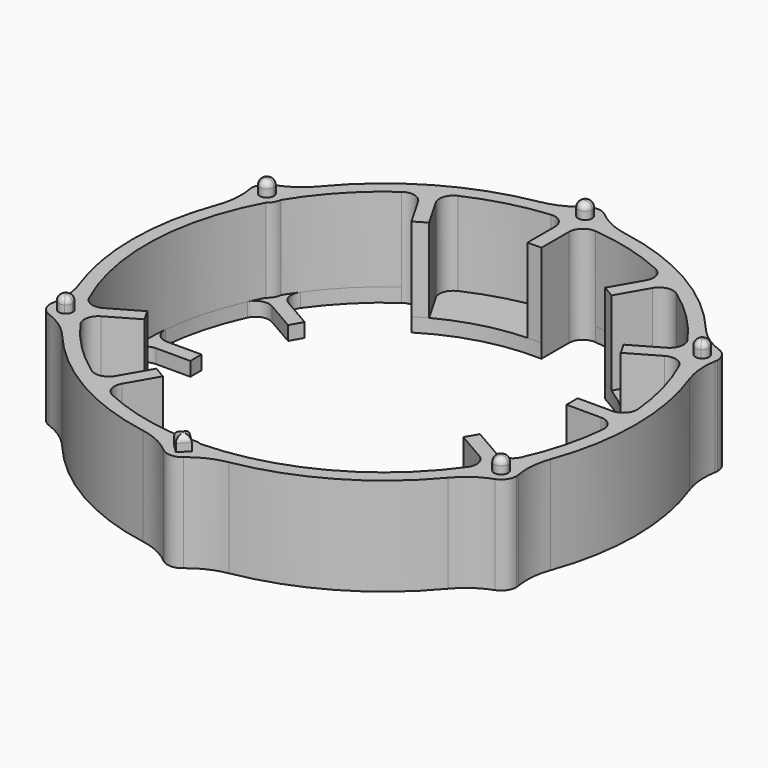
from build123d import *

# Parameters (mm, degrees)
F1_R         = 18
F1_R_2       = 17
F2_DEPTH     = 7
F3_DEPTH     = 7
F4_DEPTH     = 1
F6_DEPTH     = 7
F7_R         = 1
F8_R         = 5
F9_DEPTH     = 8
F10_R        = 0.44999
F11_DEPTH    = 1.8
F12_R        = 13.47
F13_DEPTH    = 1
F14_DEPTH    = 1
F15_T1_DEPTH = 1
F15_T3_DEPTH = 3.7395798703


# Not quite as in the source:
# - a fillet or chamfer that OpenCascade refuses, or shapes differently, is made with other operations: its cross-section is extruded or revolved along the edge and cut away or added
# - a fillet or chamfer is up to 0.001 mm smaller than in the source, because OpenCascade refuses the exact size


with BuildPart() as f2:
    # F1 (on Top) → F2 (new body)
    with BuildSketch(Plane.XY):
        Circle(F1_R)
        Circle(F1_R_2, mode=Mode.SUBTRACT)
    extrude(amount=F2_DEPTH)

    # F0 (on Top) → F3 (join)
    with BuildSketch(Plane.XY):
        with BuildLine():
            Line((7.1633711619, 11.4073228059), (8.9293354359, 14.4660626528))
            ThreePointArc((8.9293354359, 14.4660626528), (8.5, 14.7224318643), (8.0633100321, 14.9660626528))
            Line((8.0633100321, 14.9660626528), (6.2973457581, 11.9073228059))
            ThreePointArc((6.2973457581, 11.9073228059), (6.735, 11.665362189), (7.1633711619, 11.4073228059))
        make_face()
        with BuildLine():
            ThreePointArc((17, 0), (16.9981612676, 0.2500270431), (16.992645468, 0.5))
            Line((16.992645468, 0.5), (13.46071692, 0.5))
            ThreePointArc((13.46071692, 0.5), (13.46767903, 0.2500430841), (13.47, 0))
            ThreePointArc((13.47, 0), (13.46767903, -0.2500430841), (13.46071692, -0.5))
            Line((13.46071692, -0.5), (16.992645468, -0.5))
            ThreePointArc((16.992645468, -0.5), (16.9981612676, -0.2500270431), (17, 0))
        make_face()
        with BuildLine():
            ThreePointArc((-14.9660626528, -8.0633100321), (-14.7224318643, -8.5), (-14.4660626528, -8.9293354359))
            Line((-14.4660626528, -8.9293354359), (-11.4073228059, -7.1633711619))
            ThreePointArc((-11.4073228059, -7.1633711619), (-11.665362189, -6.735), (-11.9073228059, -6.2973457581))
            Line((-11.9073228059, -6.2973457581), (-14.9660626528, -8.0633100321))
        make_face()
        with BuildLine():
            Line((-6.2973457581, 11.9073228059), (-8.0633100321, 14.9660626528))
            ThreePointArc((-8.0633100321, 14.9660626528), (-8.5, 14.7224318643), (-8.9293354359, 14.4660626528))
            Line((-8.9293354359, 14.4660626528), (-7.1633711619, 11.4073228059))
            ThreePointArc((-7.1633711619, 11.4073228059), (-6.735, 11.665362189), (-6.2973457581, 11.9073228059))
        make_face()
        with BuildLine():
            Line((0.5, 13.46071692), (0.5, 16.992645468))
            ThreePointArc((0.5, 16.992645468), (0, 17), (-0.5, 16.992645468))
            Line((-0.5, 16.992645468), (-0.5, 13.46071692))
            ThreePointArc((-0.5, 13.46071692), (0, 13.47), (0.5, 13.46071692))
        make_face()
        with BuildLine():
            Line((11.9073228059, 6.2973457581), (14.9660626528, 8.0633100321))
            ThreePointArc((14.9660626528, 8.0633100321), (14.7224318643, 8.5), (14.4660626528, 8.9293354359))
            Line((14.4660626528, 8.9293354359), (11.4073228059, 7.1633711619))
            ThreePointArc((11.4073228059, 7.1633711619), (11.665362189, 6.735), (11.9073228059, 6.2973457581))
        make_face()
        with BuildLine():
            ThreePointArc((14.4660626528, -8.9293354359), (14.7224318643, -8.5), (14.9660626528, -8.0633100321))
            Line((14.9660626528, -8.0633100321), (11.9073228059, -6.2973457581))
            ThreePointArc((11.9073228059, -6.2973457581), (11.665362189, -6.735), (11.4073228059, -7.1633711619))
            Line((11.4073228059, -7.1633711619), (14.4660626528, -8.9293354359))
        make_face()
        with BuildLine():
            ThreePointArc((-8.9293354359, -14.4660626528), (-8.5, -14.7224318643), (-8.0633100321, -14.9660626528))
            Line((-8.0633100321, -14.9660626528), (-6.2973457581, -11.9073228059))
            ThreePointArc((-6.2973457581, -11.9073228059), (-6.735, -11.665362189), (-7.1633711619, -11.4073228059))
            Line((-7.1633711619, -11.4073228059), (-8.9293354359, -14.4660626528))
        make_face()
    extrude(amount=F3_DEPTH)

    # F1 (on Top) → F4 (join)
    with BuildSketch(Plane.XY):
        Circle(F1_R)
        Circle(F1_R_2, mode=Mode.SUBTRACT)
        Circle(F1_R_2)
    extrude(amount=F4_DEPTH)

    # F5 (on Top) → F6 (join)
    with BuildSketch(Plane.XY):
        with BuildLine():
            ThreePointArc((-14.4884572681, 9), (-14.6275367743, 9.5353800561), (-15.0096060035, 9.935377578))
            ThreePointArc((-15.0096060035, 9.935377578), (-15.1731450826, 9.6837837802), (-15.3324673166, 9.4294987133))
            ThreePointArc((-15.3324673166, 9.4294987133), (-15.153718855, 9.2469868663), (-15.0884572681, 9))
            ThreePointArc((-15.0884572681, 9), (-15.3354561915, 8.5687338928), (-15.832419089, 8.5635568422))
            ThreePointArc((-15.832419089, 8.5635568422), (-15.9729752997, 8.2984372068), (-16.1090923805, 8.0310113108))
            ThreePointArc((-16.1090923805, 8.0310113108), (-15.0239657375, 8.0558870238), (-14.4884572681, 9))
        make_face()
        with BuildLine():
            ThreePointArc((-15.3324673166, 9.4294987133), (-15.1731450826, 9.6837837802), (-15.0096060035, 9.935377578))
            ThreePointArc((-15.0096060035, 9.935377578), (-16.5410852123, 9.55), (-16.1090923805, 8.0310113108))
            ThreePointArc((-16.1090923805, 8.0310113108), (-15.9729752997, 8.2984372068), (-15.832419089, 8.5635568422))
            ThreePointArc((-15.832419089, 8.5635568422), (-16.02146997, 9.25), (-15.3324673166, 9.4294987133))
        make_face()
        with BuildLine():
            ThreePointArc((-1.099486377, 17.9663888889), (0, 16.9), (1.099486377, 17.9663888889))
            ThreePointArc((1.099486377, 17.9663888889), (0.7998302171, 17.982220987), (0.4999517724, 17.9930555556))
            ThreePointArc((0.4999517724, 17.9930555556), (0, 17.5), (-0.4999517724, 17.9930555556))
            ThreePointArc((-0.4999517724, 17.9930555556), (-0.7998302171, 17.982220987), (-1.099486377, 17.9663888889))
        make_face()
        with BuildLine():
            ThreePointArc((0.4999517724, 17.9930555556), (0.7998302171, 17.982220987), (1.099486377, 17.9663888889))
            ThreePointArc((1.099486377, 17.9663888889), (1.0998715868, 17.9831924823), (1.1, 18))
            ThreePointArc((1.1, 18), (-0.0168075177, 19.0998715868), (-1.099486377, 17.9663888889))
            ThreePointArc((-1.099486377, 17.9663888889), (-0.7998302171, 17.982220987), (-0.4999517724, 17.9930555556))
            ThreePointArc((-0.4999517724, 17.9930555556), (-0.003472306, 18.4999879429), (0.5, 18))
            ThreePointArc((0.5, 18), (0.4999879429, 17.996527694), (0.4999517724, 17.9930555556))
        make_face()
        with BuildLine():
            ThreePointArc((15.832419089, 8.5635568422), (15.9729752997, 8.2984372068), (16.1090923805, 8.0310113108))
            ThreePointArc((16.1090923805, 8.0310113108), (16.5325702443, 8.4355084694), (16.6884572681, 9))
            ThreePointArc((16.6884572681, 9), (16.1238373242, 9.9609204939), (15.0096060035, 9.935377578))
            ThreePointArc((15.0096060035, 9.935377578), (15.1731450826, 9.6837837802), (15.3324673166, 9.4294987133))
            ThreePointArc((15.3324673166, 9.4294987133), (15.8354441344, 9.4347384132), (16.0884572681, 9))
            ThreePointArc((16.0884572681, 9), (16.0197233753, 8.7469989234), (15.832419089, 8.5635568422))
        make_face()
        with BuildLine():
            ThreePointArc((15.0096060035, 9.935377578), (14.635829324, 8.45), (16.1090923805, 8.0310113108))
            ThreePointArc((16.1090923805, 8.0310113108), (15.9729752997, 8.2984372068), (15.832419089, 8.5635568422))
            ThreePointArc((15.832419089, 8.5635568422), (15.1554445662, 8.75), (15.3324673166, 9.4294987133))
            ThreePointArc((15.3324673166, 9.4294987133), (15.1731450826, 9.6837837802), (15.0096060035, 9.935377578))
        make_face()
        with BuildLine():
            ThreePointArc((-15.3324673166, -9.4294987133), (-15.1731450826, -9.6837837802), (-15.0096060035, -9.935377578))
            ThreePointArc((-15.0096060035, -9.935377578), (-14.6275367743, -9.5353800561), (-14.4884572681, -9))
            ThreePointArc((-14.4884572681, -9), (-15.0239657375, -8.0558870238), (-16.1090923805, -8.0310113108))
            ThreePointArc((-16.1090923805, -8.0310113108), (-15.9729752997, -8.2984372068), (-15.832419089, -8.5635568422))
            ThreePointArc((-15.832419089, -8.5635568422), (-15.3354561915, -8.5687338928), (-15.0884572681, -9))
            ThreePointArc((-15.0884572681, -9), (-15.153718855, -9.2469868663), (-15.3324673166, -9.4294987133))
        make_face()
        with BuildLine():
            ThreePointArc((-16.1090923805, -8.0310113108), (-16.5410852123, -9.55), (-15.0096060035, -9.935377578))
            ThreePointArc((-15.0096060035, -9.935377578), (-15.1731450826, -9.6837837802), (-15.3324673166, -9.4294987133))
            ThreePointArc((-15.3324673166, -9.4294987133), (-16.02146997, -9.25), (-15.832419089, -8.5635568422))
            ThreePointArc((-15.832419089, -8.5635568422), (-15.9729752997, -8.2984372068), (-16.1090923805, -8.0310113108))
        make_face()
        with BuildLine():
            ThreePointArc((0.6255239257, -17.9891278226), (0.8625800837, -17.9793202207), (1.099486377, -17.9663888889))
            ThreePointArc((1.099486377, -17.9663888889), (0, -16.9), (-1.099486377, -17.9663888889))
            ThreePointArc((-1.099486377, -17.9663888889), (-0.8625800837, -17.9793202207), (-0.6255239257, -17.9891278226))
            Line((-0.6255239257, -17.9891278226), (0, -17.3636038969))
            Line((0, -17.3636038969), (0.6255239257, -17.9891278226))
        make_face()
        with BuildLine():
            ThreePointArc((1.1, -18), (1.0998715868, -17.9831924823), (1.099486377, -17.9663888889))
            ThreePointArc((1.099486377, -17.9663888889), (0.8625800837, -17.9793202207), (0.6255239257, -17.9891278226))
            Line((0.6255239257, -17.9891278226), (0.6363961031, -18))
            Line((0.6363961031, -18), (0, -18.6363961031))
            Line((0, -18.6363961031), (-0.6363961031, -18))
            Line((-0.6363961031, -18), (-0.6255239257, -17.9891278226))
            ThreePointArc((-0.6255239257, -17.9891278226), (-0.8625800837, -17.9793202207), (-1.099486377, -17.9663888889))
            ThreePointArc((-1.099486377, -17.9663888889), (-0.0168075177, -19.0998715868), (1.1, -18))
        make_face()
        with BuildLine():
            ThreePointArc((16.6884572681, -9), (16.5325702443, -8.4355084694), (16.1090923805, -8.0310113108))
            ThreePointArc((16.1090923805, -8.0310113108), (15.9729752997, -8.2984372068), (15.832419089, -8.5635568422))
            ThreePointArc((15.832419089, -8.5635568422), (16.0197233753, -8.7469989234), (16.0884572681, -9))
            ThreePointArc((16.0884572681, -9), (15.8354441344, -9.4347384132), (15.3324673166, -9.4294987133))
            ThreePointArc((15.3324673166, -9.4294987133), (15.1731450826, -9.6837837802), (15.0096060035, -9.935377578))
            ThreePointArc((15.0096060035, -9.935377578), (16.1238373242, -9.9609204939), (16.6884572681, -9))
        make_face()
        with BuildLine():
            ThreePointArc((15.832419089, -8.5635568422), (15.9729752997, -8.2984372068), (16.1090923805, -8.0310113108))
            ThreePointArc((16.1090923805, -8.0310113108), (14.635829324, -8.45), (15.0096060035, -9.935377578))
            ThreePointArc((15.0096060035, -9.935377578), (15.1731450826, -9.6837837802), (15.3324673166, -9.4294987133))
            ThreePointArc((15.3324673166, -9.4294987133), (15.1554445662, -8.75), (15.832419089, -8.5635568422))
        make_face()
        with BuildLine():
            ThreePointArc((-15.0884572681, 9), (-15.153718855, 9.2469868663), (-15.3324673166, 9.4294987133))
            ThreePointArc((-15.3324673166, 9.4294987133), (-15.5884572681, 9), (-15.832419089, 8.5635568422))
            ThreePointArc((-15.832419089, 8.5635568422), (-15.3354561915, 8.5687338928), (-15.0884572681, 9))
        make_face()
        with BuildLine():
            ThreePointArc((-15.832419089, 8.5635568422), (-15.5884572681, 9), (-15.3324673166, 9.4294987133))
            ThreePointArc((-15.3324673166, 9.4294987133), (-16.02146997, 9.25), (-15.832419089, 8.5635568422))
        make_face()
        with BuildLine():
            ThreePointArc((-0.4999517724, 17.9930555556), (0, 18), (0.4999517724, 17.9930555556))
            ThreePointArc((0.4999517724, 17.9930555556), (0.4999879429, 17.996527694), (0.5, 18))
            ThreePointArc((0.5, 18), (-0.003472306, 18.4999879429), (-0.4999517724, 17.9930555556))
        make_face()
        with BuildLine():
            ThreePointArc((-0.4999517724, 17.9930555556), (0, 17.5), (0.4999517724, 17.9930555556))
            ThreePointArc((0.4999517724, 17.9930555556), (0, 18), (-0.4999517724, 17.9930555556))
        make_face()
        with BuildLine():
            ThreePointArc((15.3324673166, 9.4294987133), (15.5884572681, 9), (15.832419089, 8.5635568422))
            ThreePointArc((15.832419089, 8.5635568422), (16.0197233753, 8.7469989234), (16.0884572681, 9))
            ThreePointArc((16.0884572681, 9), (15.8354441344, 9.4347384132), (15.3324673166, 9.4294987133))
        make_face()
        with BuildLine():
            ThreePointArc((15.3324673166, 9.4294987133), (15.1554445662, 8.75), (15.832419089, 8.5635568422))
            ThreePointArc((15.832419089, 8.5635568422), (15.5884572681, 9), (15.3324673166, 9.4294987133))
        make_face()
        with BuildLine():
            ThreePointArc((16.0884572681, -9), (16.0197233753, -8.7469989234), (15.832419089, -8.5635568422))
            ThreePointArc((15.832419089, -8.5635568422), (15.5884572681, -9), (15.3324673166, -9.4294987133))
            ThreePointArc((15.3324673166, -9.4294987133), (15.8354441344, -9.4347384132), (16.0884572681, -9))
        make_face()
        with BuildLine():
            ThreePointArc((15.3324673166, -9.4294987133), (15.5884572681, -9), (15.832419089, -8.5635568422))
            ThreePointArc((15.832419089, -8.5635568422), (15.1554445662, -8.75), (15.3324673166, -9.4294987133))
        make_face()
        with BuildLine():
            Line((0.6363961031, -18), (0.6255239257, -17.9891278226))
            ThreePointArc((0.6255239257, -17.9891278226), (0, -18), (-0.6255239257, -17.9891278226))
            Line((-0.6255239257, -17.9891278226), (-0.6363961031, -18))
            Line((-0.6363961031, -18), (0, -18.6363961031))
            Line((0, -18.6363961031), (0.6363961031, -18))
        make_face()
        with BuildLine():
            ThreePointArc((-15.832419089, -8.5635568422), (-16.02146997, -9.25), (-15.3324673166, -9.4294987133))
            ThreePointArc((-15.3324673166, -9.4294987133), (-15.5884572681, -9), (-15.832419089, -8.5635568422))
        make_face()
        with BuildLine():
            ThreePointArc((-15.832419089, -8.5635568422), (-15.5884572681, -9), (-15.3324673166, -9.4294987133))
            ThreePointArc((-15.3324673166, -9.4294987133), (-15.153718855, -9.2469868663), (-15.0884572681, -9))
            ThreePointArc((-15.0884572681, -9), (-15.3354561915, -8.5687338928), (-15.832419089, -8.5635568422))
        make_face()
        with BuildLine():
            ThreePointArc((-0.6255239257, -17.9891278226), (0, -18), (0.6255239257, -17.9891278226))
            Line((0.6255239257, -17.9891278226), (0, -17.3636038969))
            Line((0, -17.3636038969), (-0.6255239257, -17.9891278226))
        make_face()
    extrude(amount=F6_DEPTH)

    # F7
    f7_edges = [f2.edges().sort_by_distance(p)[0] for p in [
        (0.5, 16.992645, 4),
        (-8.929335, -14.466063, 4),
        (-14.966063, -8.06331, 4),
        (16.992645, 0.5, 4),
        (-8.06331, 14.966063, 4),
        (14.966063, -8.06331, 4),
        (-0.5, 16.992645, 4),
        (8.06331, 14.966063, 4),
        (14.466063, 8.929335, 4),
        (16.992645, -0.5, 4),
        (14.466063, -8.929335, 4),
        (-8.929335, 14.466063, 4),
        (-14.466063, -8.929335, 4),
        (-8.06331, -14.966063, 4),
        (14.966063, 8.06331, 4),
        (8.929335, 14.466063, 4),
    ]]
    fillet(f7_edges, radius=F7_R)

    # F8 (call 1 of 12: OpenCascade refuses the feature's edges together)
    f8_edges = [f2.edges().sort_by_distance(p)[0] for p in [
        (-16.109092, 8.031011, 3.5),
    ]]
    fillet(f8_edges, radius=F8_R)

    # F8#2 (call 2 of 12)
    f8_2_edges = [f2.edges().sort_by_distance(p)[0] for p in [
        (-15.009606, 9.935378, 3.5),
    ]]
    fillet(f8_2_edges, radius=F8_R)

    # F8#3 (call 3 of 12)
    f8_3_edges = [f2.edges().sort_by_distance(p)[0] for p in [
        (-1.099486, 17.966389, 3.5),
    ]]
    fillet(f8_3_edges, radius=F8_R)

    # F8#4 (call 4 of 12)
    f8_4_edges = [f2.edges().sort_by_distance(p)[0] for p in [
        (1.099486, 17.966389, 3.5),
    ]]
    fillet(f8_4_edges, radius=F8_R)

    # F8#5 (call 5 of 12)
    f8_5_edges = [f2.edges().sort_by_distance(p)[0] for p in [
        (-15.009606, -9.935378, 3.5),
    ]]
    fillet(f8_5_edges, radius=F8_R)

    # F8#6 (call 6 of 12)
    f8_6_edges = [f2.edges().sort_by_distance(p)[0] for p in [
        (-16.109092, -8.031011, 3.5),
    ]]
    fillet(f8_6_edges, radius=F8_R)

    # F8#7 (call 7 of 12)
    f8_7_edges = [f2.edges().sort_by_distance(p)[0] for p in [
        (1.099486, -17.966389, 3.5),
    ]]
    fillet(f8_7_edges, radius=F8_R)

    # F8#8 (call 8 of 12)
    f8_8_edges = [f2.edges().sort_by_distance(p)[0] for p in [
        (-1.099486, -17.966389, 3.5),
    ]]
    fillet(f8_8_edges, radius=F8_R)

    # F8#10 (call 9 of 12)
    f8_10_edges = [f2.edges().sort_by_distance(p)[0] for p in [
        (15.009606, -9.935378, 3.5),
    ]]
    fillet(f8_10_edges, radius=F8_R)

    # F8#11 (call 10 of 12)
    f8_11_edges = [f2.edges().sort_by_distance(p)[0] for p in [
        (16.109092, 8.031011, 3.5),
    ]]
    fillet(f8_11_edges, radius=F8_R)

    # F8#12 (call 11 of 12)
    f8_12_edges = [f2.edges().sort_by_distance(p)[0] for p in [
        (15.009606, 9.935378, 3.5),
    ]]
    fillet(f8_12_edges, radius=F8_R)

    # F8#9 (call 12 of 12)
    f8_9_edges = [f2.edges().sort_by_distance(p)[0] for p in [
        (16.109092, -8.031011, 3.5),
    ]]
    fillet(f8_9_edges, radius=F8_R)

    # F5 (on Top) → F9 (join)
    with BuildSketch(Plane.XY):
        with BuildLine():
            ThreePointArc((-15.832419089, 8.5635568422), (-15.5884572681, 9), (-15.3324673166, 9.4294987133))
            ThreePointArc((-15.3324673166, 9.4294987133), (-16.02146997, 9.25), (-15.832419089, 8.5635568422))
        make_face()
        with BuildLine():
            ThreePointArc((-15.0884572681, 9), (-15.153718855, 9.2469868663), (-15.3324673166, 9.4294987133))
            ThreePointArc((-15.3324673166, 9.4294987133), (-15.5884572681, 9), (-15.832419089, 8.5635568422))
            ThreePointArc((-15.832419089, 8.5635568422), (-15.3354561915, 8.5687338928), (-15.0884572681, 9))
        make_face()
        with BuildLine():
            ThreePointArc((-0.4999517724, 17.9930555556), (0, 18), (0.4999517724, 17.9930555556))
            ThreePointArc((0.4999517724, 17.9930555556), (0.4999879429, 17.996527694), (0.5, 18))
            ThreePointArc((0.5, 18), (-0.003472306, 18.4999879429), (-0.4999517724, 17.9930555556))
        make_face()
        with BuildLine():
            ThreePointArc((-0.4999517724, 17.9930555556), (0, 17.5), (0.4999517724, 17.9930555556))
            ThreePointArc((0.4999517724, 17.9930555556), (0, 18), (-0.4999517724, 17.9930555556))
        make_face()
        with BuildLine():
            ThreePointArc((15.3324673166, 9.4294987133), (15.1554445662, 8.75), (15.832419089, 8.5635568422))
            ThreePointArc((15.832419089, 8.5635568422), (15.5884572681, 9), (15.3324673166, 9.4294987133))
        make_face()
        with BuildLine():
            ThreePointArc((15.3324673166, 9.4294987133), (15.5884572681, 9), (15.832419089, 8.5635568422))
            ThreePointArc((15.832419089, 8.5635568422), (16.0197233753, 8.7469989234), (16.0884572681, 9))
            ThreePointArc((16.0884572681, 9), (15.8354441344, 9.4347384132), (15.3324673166, 9.4294987133))
        make_face()
        with BuildLine():
            ThreePointArc((15.3324673166, -9.4294987133), (15.5884572681, -9), (15.832419089, -8.5635568422))
            ThreePointArc((15.832419089, -8.5635568422), (15.1554445662, -8.75), (15.3324673166, -9.4294987133))
        make_face()
        with BuildLine():
            ThreePointArc((16.0884572681, -9), (16.0197233753, -8.7469989234), (15.832419089, -8.5635568422))
            ThreePointArc((15.832419089, -8.5635568422), (15.5884572681, -9), (15.3324673166, -9.4294987133))
            ThreePointArc((15.3324673166, -9.4294987133), (15.8354441344, -9.4347384132), (16.0884572681, -9))
        make_face()
        with BuildLine():
            Line((0.6363961031, -18), (0.6255239257, -17.9891278226))
            ThreePointArc((0.6255239257, -17.9891278226), (0, -18), (-0.6255239257, -17.9891278226))
            Line((-0.6255239257, -17.9891278226), (-0.6363961031, -18))
            Line((-0.6363961031, -18), (0, -18.6363961031))
            Line((0, -18.6363961031), (0.6363961031, -18))
        make_face()
        with BuildLine():
            ThreePointArc((-0.6255239257, -17.9891278226), (0, -18), (0.6255239257, -17.9891278226))
            Line((0.6255239257, -17.9891278226), (0, -17.3636038969))
            Line((0, -17.3636038969), (-0.6255239257, -17.9891278226))
        make_face()
        with BuildLine():
            ThreePointArc((-15.832419089, -8.5635568422), (-16.02146997, -9.25), (-15.3324673166, -9.4294987133))
            ThreePointArc((-15.3324673166, -9.4294987133), (-15.5884572681, -9), (-15.832419089, -8.5635568422))
        make_face()
        with BuildLine():
            ThreePointArc((-15.832419089, -8.5635568422), (-15.5884572681, -9), (-15.3324673166, -9.4294987133))
            ThreePointArc((-15.3324673166, -9.4294987133), (-15.153718855, -9.2469868663), (-15.0884572681, -9))
            ThreePointArc((-15.0884572681, -9), (-15.3354561915, -8.5687338928), (-15.832419089, -8.5635568422))
        make_face()
    extrude(amount=F9_DEPTH)

    # F10 (radius 0.45 in the source; OpenCascade refuses exactly that, so slightly less here)
    f10_edges = [f2.edges().sort_by_distance(p)[0] for p in [
        (-15.844447, -8.570501, 8),
        (-15.344495, 9.436443, 8),
        (0.499952, 18.006944, 8),
        (15.344495, 9.436443, 8),
        (15.844447, -8.570501, 8),
        (0.318198, -17.681802, 8),
        (-0.318198, -18.318198, 8),
        (0.318198, -18.318198, 8),
        (-0.318198, -17.681802, 8),
    ]]
    fillet(f10_edges, radius=F10_R)

    # F5 (on Top) → F11 (cut)
    with BuildSketch(Plane.XY):
        with BuildLine():
            ThreePointArc((-15.832419089, -8.5635568422), (-16.02146997, -9.25), (-15.3324673166, -9.4294987133))
            ThreePointArc((-15.3324673166, -9.4294987133), (-15.5884572681, -9), (-15.832419089, -8.5635568422))
        make_face()
        with BuildLine():
            ThreePointArc((-15.832419089, -8.5635568422), (-15.5884572681, -9), (-15.3324673166, -9.4294987133))
            ThreePointArc((-15.3324673166, -9.4294987133), (-15.153718855, -9.2469868663), (-15.0884572681, -9))
            ThreePointArc((-15.0884572681, -9), (-15.3354561915, -8.5687338928), (-15.832419089, -8.5635568422))
        make_face()
        with BuildLine():
            Line((0.6363961031, -18), (0.6255239257, -17.9891278226))
            ThreePointArc((0.6255239257, -17.9891278226), (0, -18), (-0.6255239257, -17.9891278226))
            Line((-0.6255239257, -17.9891278226), (-0.6363961031, -18))
            Line((-0.6363961031, -18), (0, -18.6363961031))
            Line((0, -18.6363961031), (0.6363961031, -18))
        make_face()
        with BuildLine():
            ThreePointArc((-0.6255239257, -17.9891278226), (0, -18), (0.6255239257, -17.9891278226))
            Line((0.6255239257, -17.9891278226), (0, -17.3636038969))
            Line((0, -17.3636038969), (-0.6255239257, -17.9891278226))
        make_face()
        with BuildLine():
            ThreePointArc((15.3324673166, -9.4294987133), (15.5884572681, -9), (15.832419089, -8.5635568422))
            ThreePointArc((15.832419089, -8.5635568422), (15.1554445662, -8.75), (15.3324673166, -9.4294987133))
        make_face()
        with BuildLine():
            ThreePointArc((16.0884572681, -9), (16.0197233753, -8.7469989234), (15.832419089, -8.5635568422))
            ThreePointArc((15.832419089, -8.5635568422), (15.5884572681, -9), (15.3324673166, -9.4294987133))
            ThreePointArc((15.3324673166, -9.4294987133), (15.8354441344, -9.4347384132), (16.0884572681, -9))
        make_face()
        with BuildLine():
            ThreePointArc((15.3324673166, 9.4294987133), (15.1554445662, 8.75), (15.832419089, 8.5635568422))
            ThreePointArc((15.832419089, 8.5635568422), (15.5884572681, 9), (15.3324673166, 9.4294987133))
        make_face()
        with BuildLine():
            ThreePointArc((15.3324673166, 9.4294987133), (15.5884572681, 9), (15.832419089, 8.5635568422))
            ThreePointArc((15.832419089, 8.5635568422), (16.0197233753, 8.7469989234), (16.0884572681, 9))
            ThreePointArc((16.0884572681, 9), (15.8354441344, 9.4347384132), (15.3324673166, 9.4294987133))
        make_face()
        with BuildLine():
            ThreePointArc((-0.4999517724, 17.9930555556), (0, 17.5), (0.4999517724, 17.9930555556))
            ThreePointArc((0.4999517724, 17.9930555556), (0, 18), (-0.4999517724, 17.9930555556))
        make_face()
        with BuildLine():
            ThreePointArc((-0.4999517724, 17.9930555556), (0, 18), (0.4999517724, 17.9930555556))
            ThreePointArc((0.4999517724, 17.9930555556), (0.4999879429, 17.996527694), (0.5, 18))
            ThreePointArc((0.5, 18), (-0.003472306, 18.4999879429), (-0.4999517724, 17.9930555556))
        make_face()
        with BuildLine():
            ThreePointArc((-15.832419089, 8.5635568422), (-15.5884572681, 9), (-15.3324673166, 9.4294987133))
            ThreePointArc((-15.3324673166, 9.4294987133), (-16.02146997, 9.25), (-15.832419089, 8.5635568422))
        make_face()
        with BuildLine():
            ThreePointArc((-15.0884572681, 9), (-15.153718855, 9.2469868663), (-15.3324673166, 9.4294987133))
            ThreePointArc((-15.3324673166, 9.4294987133), (-15.5884572681, 9), (-15.832419089, 8.5635568422))
            ThreePointArc((-15.832419089, 8.5635568422), (-15.3354561915, 8.5687338928), (-15.0884572681, 9))
        make_face()
    extrude(amount=F11_DEPTH, mode=Mode.SUBTRACT)

    # F12 (on Top) → F13 (cut)
    with BuildSketch(Plane.XY):
        Circle(F12_R)
    extrude(amount=F13_DEPTH, mode=Mode.SUBTRACT)

    # F0 (on Top) → F14 (cut)
    with BuildSketch(Plane.XY):
        with BuildLine():
            ThreePointArc((0.5, -16.992645468), (4.3999237667, -16.4207390469), (8.0633100321, -14.9660626528))
            Line((8.0633100321, -14.9660626528), (6.2973457581, -11.9073228059))
            ThreePointArc((6.2973457581, -11.9073228059), (3.4862925375, -13.0110208801), (0.5, -13.46071692))
            Line((0.5, -13.46071692), (0.5, -16.992645468))
        make_face()
        with BuildLine():
            ThreePointArc((14.9660626528, -8.0633100321), (16.4207390469, -4.3999237667), (16.992645468, -0.5))
            Line((16.992645468, -0.5), (13.46071692, -0.5))
            ThreePointArc((13.46071692, -0.5), (13.0110208801, -3.4862925375), (11.9073228059, -6.2973457581))
            Line((11.9073228059, -6.2973457581), (14.9660626528, -8.0633100321))
        make_face()
        with BuildLine():
            Line((13.46071692, 0.5), (16.992645468, 0.5))
            ThreePointArc((16.992645468, 0.5), (16.4207390469, 4.3999237667), (14.9660626528, 8.0633100321))
            Line((14.9660626528, 8.0633100321), (11.9073228059, 6.2973457581))
            ThreePointArc((11.9073228059, 6.2973457581), (13.0110208801, 3.4862925375), (13.46071692, 0.5))
        make_face()
        with BuildLine():
            Line((6.2973457581, 11.9073228059), (8.0633100321, 14.9660626528))
            ThreePointArc((8.0633100321, 14.9660626528), (4.3999237667, 16.4207390469), (0.5, 16.992645468))
            Line((0.5, 16.992645468), (0.5, 13.46071692))
            ThreePointArc((0.5, 13.46071692), (3.4862925375, 13.0110208801), (6.2973457581, 11.9073228059))
        make_face()
        with BuildLine():
            Line((-7.1633711619, 11.4073228059), (-8.9293354359, 14.4660626528))
            ThreePointArc((-8.9293354359, 14.4660626528), (-12.0208152802, 12.0208152802), (-14.4660626528, 8.9293354359))
            Line((-14.4660626528, 8.9293354359), (-11.4073228059, 7.1633711619))
            ThreePointArc((-11.4073228059, 7.1633711619), (-9.5247283426, 9.5247283426), (-7.1633711619, 11.4073228059))
        make_face()
        with BuildLine():
            Line((-11.9073228059, 6.2973457581), (-14.9660626528, 8.0633100321))
            ThreePointArc((-14.9660626528, 8.0633100321), (-16.4207390469, 4.3999237667), (-16.992645468, 0.5))
            Line((-16.992645468, 0.5), (-13.46071692, 0.5))
            ThreePointArc((-13.46071692, 0.5), (-13.0110208801, 3.4862925375), (-11.9073228059, 6.2973457581))
        make_face()
        with BuildLine():
            ThreePointArc((-16.992645468, -0.5), (-16.4207390469, -4.3999237667), (-14.9660626528, -8.0633100321))
            Line((-14.9660626528, -8.0633100321), (-11.9073228059, -6.2973457581))
            ThreePointArc((-11.9073228059, -6.2973457581), (-13.0110208801, -3.4862925375), (-13.46071692, -0.5))
            Line((-13.46071692, -0.5), (-16.992645468, -0.5))
        make_face()
        with BuildLine():
            ThreePointArc((-14.4660626528, -8.9293354359), (-12.0208152802, -12.0208152802), (-8.9293354359, -14.4660626528))
            Line((-8.9293354359, -14.4660626528), (-7.1633711619, -11.4073228059))
            ThreePointArc((-7.1633711619, -11.4073228059), (-9.5247283426, -9.5247283426), (-11.4073228059, -7.1633711619))
            Line((-11.4073228059, -7.1633711619), (-14.4660626528, -8.9293354359))
        make_face()
    extrude(amount=F14_DEPTH, mode=Mode.SUBTRACT)

    # F15: fillet of radius 1 on 16 edges, made by hand

    # F15_s2 → F15_t1 (join)
    with BuildSketch(Plane.XY):
        with BuildLine():
            ThreePointArc((-15.4544658902, 7.0823360588), (-14.8492412837, 7.6184442326), (-14.0453796613, 7.5317534591))
            Line((-14.0453796613, 7.5317534591), (-14.9660626528, 8.0633100321))
            ThreePointArc((-14.9660626528, 8.0633100321), (-15.2181706092, 7.57675942), (-15.4544658902, 7.0823360588))
        make_face()
        with BuildLine():
            ThreePointArc((-16.9251280922, -1.59375), (-16.669042295, -0.8268543991), (-15.9295323221, -0.5))
            Line((-15.9295323221, -0.5), (-16.992645468, -0.5))
            ThreePointArc((-16.992645468, -0.5), (-16.9677020567, -1.0474191685), (-16.9251280922, -1.59375))
        make_face()
        with BuildLine():
            ThreePointArc((-16.9251280922, 1.59375), (-16.669042295, 0.8268543991), (-15.9295323221, 0.5))
            Line((-15.9295323221, 0.5), (-16.992645468, 0.5))
            ThreePointArc((-16.992645468, 0.5), (-16.9677020567, 1.0474191685), (-16.9251280922, 1.59375))
        make_face()
        with BuildLine():
            ThreePointArc((-13.8607158902, 9.8427920334), (-14.0223868846, 9.0505980623), (-13.5453796613, 8.3977788629))
            Line((-13.5453796613, 8.3977788629), (-14.4660626528, 8.9293354359))
            ThreePointArc((-14.4660626528, 8.9293354359), (-14.1707514407, 9.3909426367), (-13.8607158902, 9.8427920334))
        make_face()
        with BuildLine():
            ThreePointArc((1.59375, -16.9251280922), (0.8268543991, -16.669042295), (0.5, -15.9295323221))
            Line((0.5, -15.9295323221), (0.5, -16.992645468))
            ThreePointArc((0.5, -16.992645468), (1.0474191685, -16.9677020567), (1.59375, -16.9251280922))
        make_face()
        with BuildLine():
            ThreePointArc((7.0823360588, -15.4544658902), (7.6184442326, -14.8492412837), (7.5317534591, -14.0453796613))
            Line((7.5317534591, -14.0453796613), (8.0633100321, -14.9660626528))
            ThreePointArc((8.0633100321, -14.9660626528), (7.57675942, -15.2181706092), (7.0823360588, -15.4544658902))
        make_face()
    extrude(amount=F15_T1_DEPTH)

    # F15_s4 → F15_t3 (join)
    with BuildSketch(Plane.XY):
        with BuildLine():
            ThreePointArc((-14.0453796613, -7.5317534591), (-14.8492412838, -7.6184442326), (-15.4544658902, -7.0823360588))
            ThreePointArc((-15.4544658902, -7.0823360588), (-15.2181706092, -7.57675942), (-14.9660626528, -8.0633100321))
            Line((-14.9660626528, -8.0633100321), (-14.0453796613, -7.5317534591))
        make_face()
        with BuildLine():
            ThreePointArc((-8.3977788629, -13.5453796613), (-9.0505980623, -14.0223868846), (-9.8427920334, -13.8607158902))
            ThreePointArc((-9.8427920334, -13.8607158902), (-9.3909426367, -14.1707514407), (-8.9293354359, -14.4660626528))
            Line((-8.9293354359, -14.4660626528), (-8.3977788629, -13.5453796613))
        make_face()
        with BuildLine():
            ThreePointArc((-13.8607158902, -9.8427920334), (-14.0223868846, -9.0505980623), (-13.5453796613, -8.3977788629))
            Line((-13.5453796613, -8.3977788629), (-14.4660626528, -8.9293354359))
            ThreePointArc((-14.4660626528, -8.9293354359), (-14.1707514407, -9.3909426367), (-13.8607158902, -9.8427920334))
        make_face()
        with BuildLine():
            ThreePointArc((-9.8427920334, 13.8607158902), (-9.0505980623, 14.0223868846), (-8.3977788629, 13.5453796613))
            Line((-8.3977788629, 13.5453796613), (-8.9293354359, 14.4660626528))
            ThreePointArc((-8.9293354359, 14.4660626528), (-9.3909426367, 14.1707514407), (-9.8427920334, 13.8607158902))
        make_face()
        with BuildLine():
            ThreePointArc((1.59375, 16.9251280922), (0.8268543991, 16.669042295), (0.5, 15.9295323221))
            Line((0.5, 15.9295323221), (0.5, 16.992645468))
            ThreePointArc((0.5, 16.992645468), (1.0474191685, 16.9677020567), (1.59375, 16.9251280922))
        make_face()
        with BuildLine():
            ThreePointArc((14.0453796613, -7.5317534591), (14.8492412838, -7.6184442326), (15.4544658902, -7.0823360588))
            ThreePointArc((15.4544658902, -7.0823360588), (15.2181706092, -7.57675942), (14.9660626528, -8.0633100321))
            Line((14.9660626528, -8.0633100321), (14.0453796613, -7.5317534591))
        make_face()
        with BuildLine():
            ThreePointArc((15.9295323221, 0.5), (16.669042295, 0.8268543991), (16.9251280922, 1.59375))
            ThreePointArc((16.9251280922, 1.59375), (16.9677020567, 1.0474191685), (16.992645468, 0.5))
            Line((16.992645468, 0.5), (15.9295323221, 0.5))
        make_face()
        with BuildLine():
            ThreePointArc((7.5317534591, 14.0453796613), (7.6184442326, 14.8492412838), (7.0823360588, 15.4544658902))
            ThreePointArc((7.0823360588, 15.4544658902), (7.57675942, 15.2181706092), (8.0633100321, 14.9660626528))
            Line((8.0633100321, 14.9660626528), (7.5317534591, 14.0453796613))
        make_face()
        with BuildLine():
            ThreePointArc((15.4544658902, 7.0823360588), (14.8492412837, 7.6184442326), (14.0453796613, 7.5317534591))
            Line((14.0453796613, 7.5317534591), (14.9660626528, 8.0633100321))
            ThreePointArc((14.9660626528, 8.0633100321), (15.2181706092, 7.57675942), (15.4544658902, 7.0823360588))
        make_face()
        with BuildLine():
            ThreePointArc((16.9251280922, -1.59375), (16.669042295, -0.8268543991), (15.9295323221, -0.5))
            Line((15.9295323221, -0.5), (16.992645468, -0.5))
            ThreePointArc((16.992645468, -0.5), (16.9677020567, -1.0474191685), (16.9251280922, -1.59375))
        make_face()
    extrude(amount=F15_T3_DEPTH)


solid = f2.part
